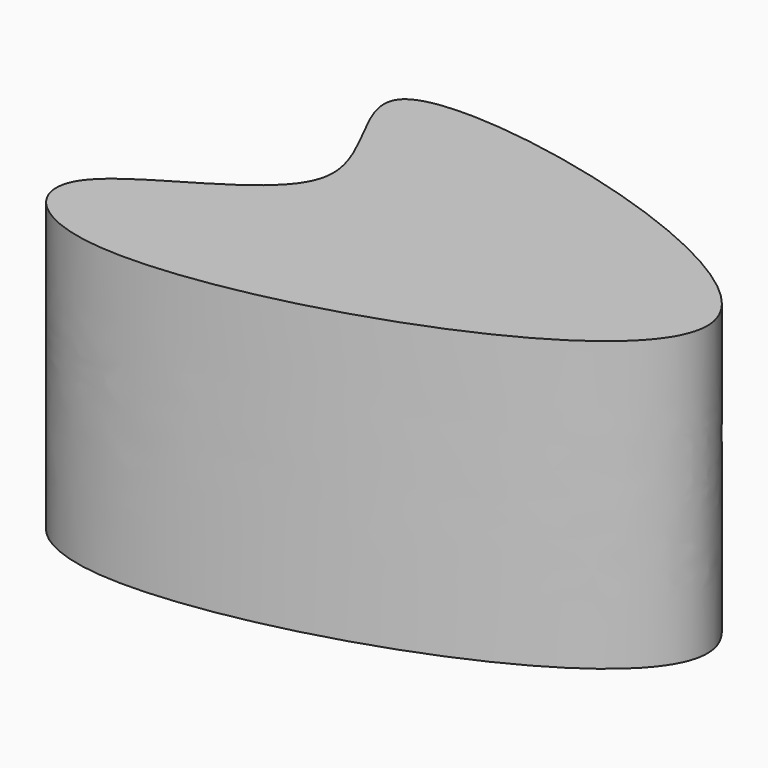
from build123d import *

# Parameters (mm, degrees)
F1_DEPTH = 44.2477241158


# Not quite as in the source:
# - the program builds the solid bodies; features that only make, move or delete a surface that nothing else refers to are left out


with BuildPart() as f1:
    # F0 (on Top) → F1 (new body)
    with BuildSketch(Plane.XY):
        with BuildLine():
            add(Edge.make_bspline(
                [(-33.4232822061, 66.9687762856), (-26.0111572837, 73.7037310164), (84.4881890479, 46.8649190871), (-40.1634909903, 3.3038282964), (-59.285551706, 29.124907217), (-14.6239266757, 41.1753797496), (-37.6215326499, 63.1540771294), (-33.4232822061, 66.9687762856)],
                knots=[0, 0, 0, 0, 0.2644896632, 0.5451255897, 0.6757023333, 0.8501922381, 1, 1, 1, 1], degree=3))
        make_face()
    extrude(amount=F1_DEPTH)


solid = f1.part
